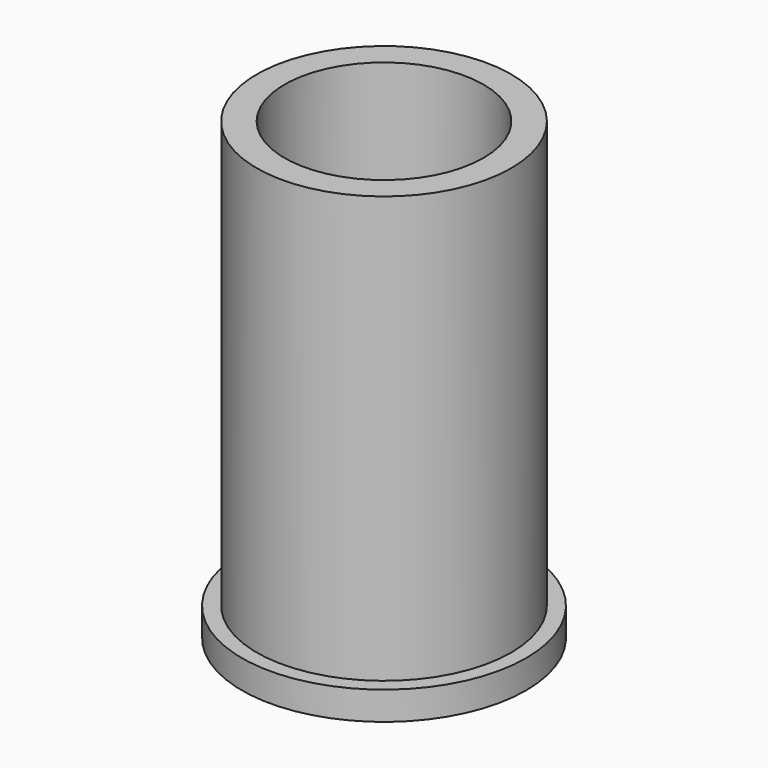
from build123d import *

# Parameters (mm, degrees)
F0_R     = 8.95
F0_R_2   = 7
F1_DEPTH = 30
F2_R     = 10
F2_R_2   = 8.95
F2_R_3   = 7
F3_DEPTH = 2


with BuildPart() as f1:
    # F0 (on Top) → F1 (new body)
    with BuildSketch(Plane.XY):
        Circle(F0_R)
        Circle(F0_R_2, mode=Mode.SUBTRACT)
    extrude(amount=F1_DEPTH)

    # F2 (on face) → F3 (join)
    with BuildSketch(Plane(origin=(0, 0, 0), x_dir=(1, 0, 0), z_dir=(0, 0, -1))):
        Circle(F2_R)
        Circle(F2_R_2, mode=Mode.SUBTRACT)
        Circle(F2_R_2)
        Circle(F2_R_3, mode=Mode.SUBTRACT)
    extrude(amount=F3_DEPTH)


solid = f1.part
